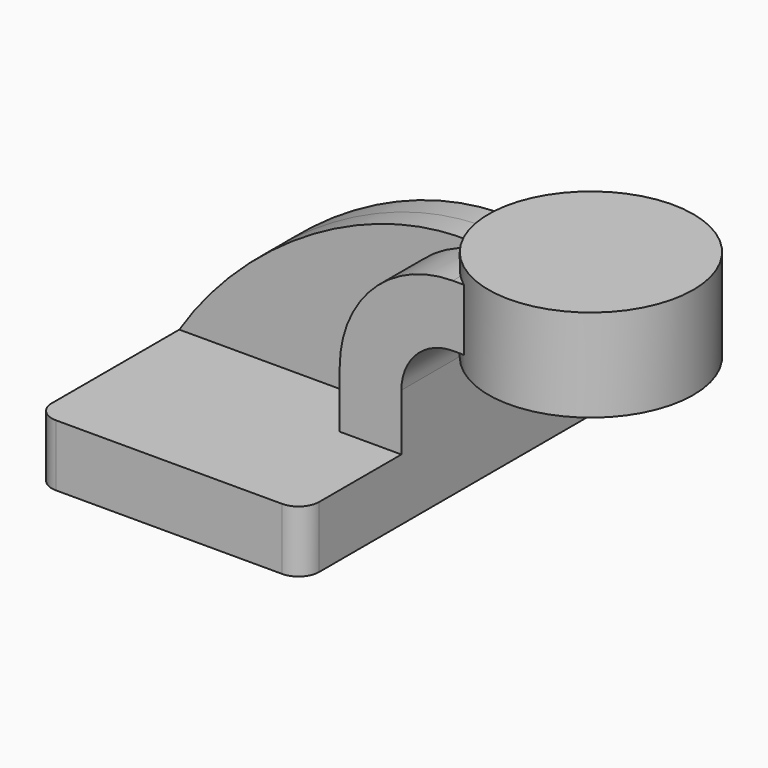
from build123d import *

# Parameters (mm, degrees)
F1_DEPTH = 63.5
F0_W     = 19.1631158481
F0_H     = 19.05
F2_DEPTH = 25.4
F3_DEPTH = 7.9375
F4_R     = 6.35


with BuildPart() as f1:
    # F0 (on Front) → F1 (new body, symmetric)
    with BuildSketch(Plane.XZ):
        Polygon((22.225, 9.525), (-41.275, 9.525), (-41.275, -9.525), (41.275, -9.525), (41.275, 9.525), align=None)
    extrude(amount=F1_DEPTH, both=True)

    # F0 (on Front) → F2 (join, symmetric)
    with BuildSketch(Plane.XZ):
        with BuildLine():
            Line((22.225, 27.0002), (22.225, 9.525))
            Line((22.225, 9.525), (41.275, 9.525))
            Line((41.275, 9.525), (41.275, 27.0002))
            ThreePointArc((41.275, 27.0002), (45.9246798487, 38.2255201513), (57.15, 42.8752))
            Line((57.15, 42.8752), (60.325, 42.8752))
            Line((60.325, 42.8752), (60.325, 61.9252))
            Line((60.325, 61.9252), (57.15, 61.9252))
            ThreePointArc((57.15, 61.9252), (32.4542956671, 51.6959043329), (22.225, 27.0002))
        make_face()
        with Locations((69.9065579241, 52.4002)):
            Rectangle(F0_W, F0_H)
    extrude(amount=F2_DEPTH, both=True)

    # F0 (on Front) → F3 (join, symmetric)
    with BuildSketch(Plane.XZ):
        with BuildLine():
            add(Edge.make_bspline(
                [(-41.275, 9.525), (-19.9898480937, 42.9106190082), (22.3848360241, 68.1215267785), (57.15, 61.9252)],
                knots=[0, 0, 0, 0, 111.5045361635, 111.5045361635, 111.5045361635, 111.5045361635], degree=3))
            Line((-41.275, 9.525), (22.225, 9.525))
            Line((22.225, 9.525), (22.225, 27.0002))
            ThreePointArc((22.225, 27.0002), (32.4542956671, 51.6959043329), (57.15, 61.9252))
        make_face()
    extrude(amount=F3_DEPTH, both=True)

    # F4
    f4_edges = [f1.edges().sort_by_distance(p)[0] for p in [
        (-41.275, -63.5, 0),
        (41.275, -63.5, 0),
        (41.275, 63.5, 0),
        (-41.275, 63.5, 0),
    ]]
    fillet(f4_edges, radius=F4_R)

    # F0 (on Front) → F5 (revolve)
    with BuildSketch(Plane.XZ):
        Polygon((79.4881158481, 66.675), (79.4881158481, 61.9252), (79.4881158481, 42.8752), (79.4881158481, 38.1), (111.125, 38.1), (111.125, 66.675), align=None)
    revolve(axis=Axis((79.4881158481, 0, 52.3875), (0, 0, 1)))


solid = f1.part
